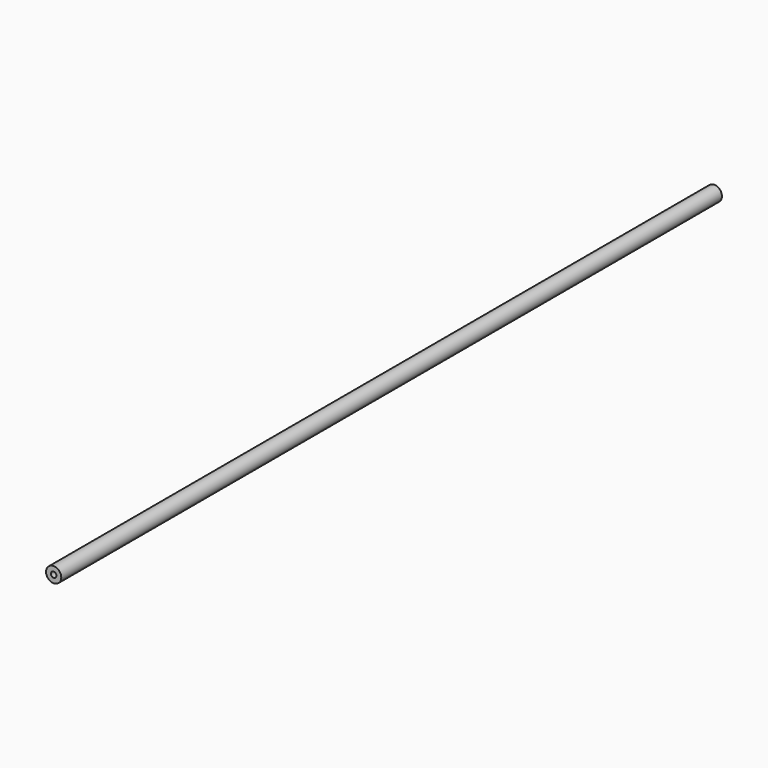
from build123d import *

# Parameters (mm, degrees)
F1_R     = 17.527805963
F1_R_2   = 6.35
F2_DEPTH = 1905


with BuildPart() as f2:
    # F1 (on Front) → F2 (new body)
    with BuildSketch(Plane.XZ):
        Circle(F1_R)
        Circle(F1_R_2, mode=Mode.SUBTRACT)
    extrude(amount=F2_DEPTH)


solid = f2.part
